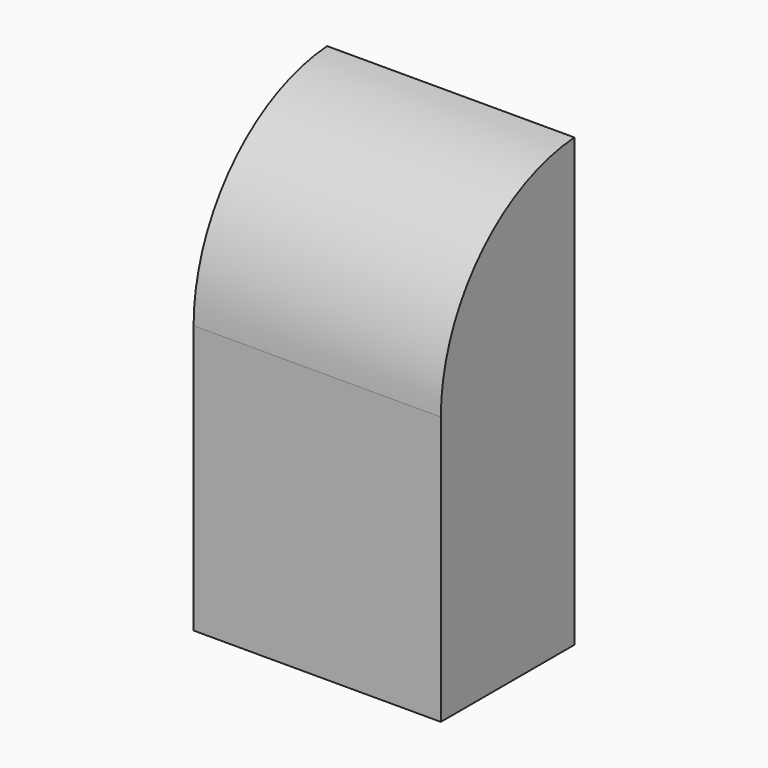
from build123d import *

# Parameters (mm, degrees)
F1_W        = 70.3014656901
F1_H        = 47.4647134542
F0_DEPTH    = 127
F2_T1_DEPTH = 323.753426802


# Not quite as in the source:
# - a fillet or chamfer that OpenCascade refuses, or shapes differently, is made with other operations: its cross-section is extruded or revolved along the edge and cut away or added


with BuildPart() as f0:
    # F1 (on Top) → F0 (new body)
    with BuildSketch(Plane.XY):
        Rectangle(F1_W, F1_H)
    extrude(amount=F0_DEPTH)

    # F2: fillet of radius 50.8 on 1 edges, made by hand

    # F2_s2 → F2_t1 (cut)
    with BuildSketch(Plane.YZ.offset(-161.876713401)):
        with BuildLine():
            ThreePointArc((-23.7323567271, 76.3096077776), (-10.0138383354, 111.0314124793), (23.7323567271, 127))
            Line((23.7323567271, 127), (-23.7323567271, 127))
            Line((-23.7323567271, 127), (-23.7323567271, 76.3096077776))
        make_face()
    extrude(amount=F2_T1_DEPTH, mode=Mode.SUBTRACT)


solid = f0.part
